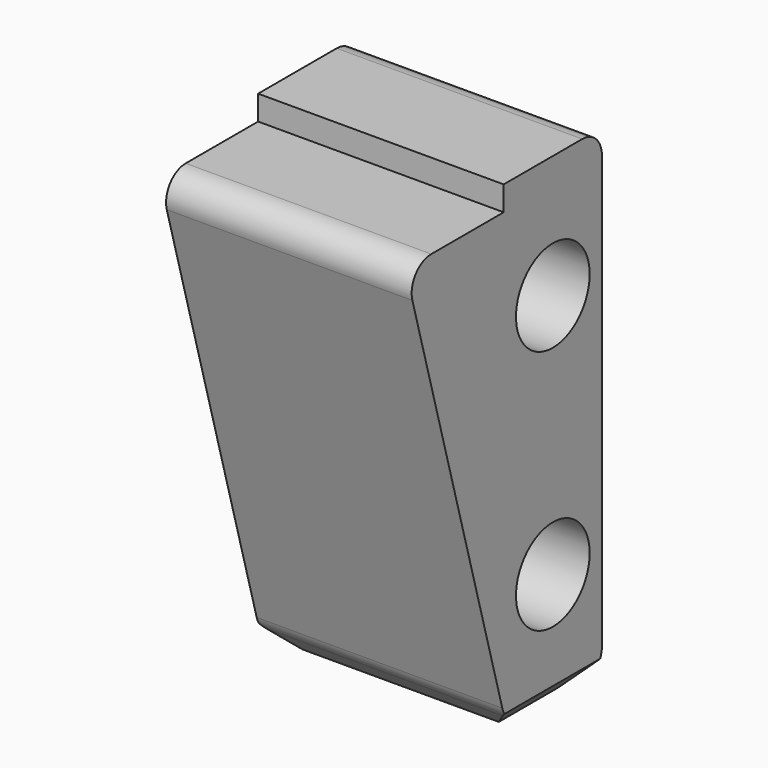
from build123d import *

# Parameters (mm, degrees)
F0_W     = 50.8
F0_H     = 101.6
F1_DEPTH = 25.4
F2_R     = 9.525
F3_DEPTH = 50.8
F4_SIZE  = 5.08
F7_DEPTH = 50.8
F8_R     = 5.08


# Not quite as in the source:
# - a feature of the source that left no trace in its solid (it failed there, or was rolled back) is left out


with BuildPart() as f1:
    # F0 (on Front) → F1 (new body)
    with BuildSketch(Plane.XZ):
        with Locations((20.7021635301, -10.4186603248)):
            Rectangle(F0_W, F0_H)
    extrude(amount=F1_DEPTH)

    # F2 (on face) → F3 (cut)
    with BuildSketch(Plane.YZ.offset(46.1021635301)):
        with Locations((-12.7, 14.9813396752)):
            Circle(F2_R)
        with Locations((-12.7, -35.8186603248)):
            Circle(F2_R)
    extrude(amount=-F3_DEPTH, mode=Mode.SUBTRACT)

    # F4
    f4_edges = [f1.edges().sort_by_distance(p)[0] for p in [
        (-4.697836, -12.7, -61.21866),
        (46.102164, -12.7, -61.21866),
        (20.702164, 0, -61.21866),
        (20.702164, -25.4, -61.21866),
    ]]
    chamfer(f4_edges, length=F4_SIZE)

    # F6 (on face) → F7 (join)
    with BuildSketch(Plane(origin=(-4.6978364699, 0, 0), x_dir=(0, -1, 0), z_dir=(-1, 0, 0))):
        Polygon((50.8, 35.3013396752), (25.4, 35.3013396752), (25.4, -56.1386603248), align=None)
    extrude(amount=-F7_DEPTH)

    # F8
    f8_edges = [f1.edges().sort_by_distance(p)[0] for p in [
        (20.702164, -50.8, 35.30134),
        (20.702164, 0, 40.38134),
        (20.702164, -25.4, -56.13866),
        (20.702164, 0, -56.13866),
    ]]
    fillet(f8_edges, radius=F8_R)


solid = f1.part
